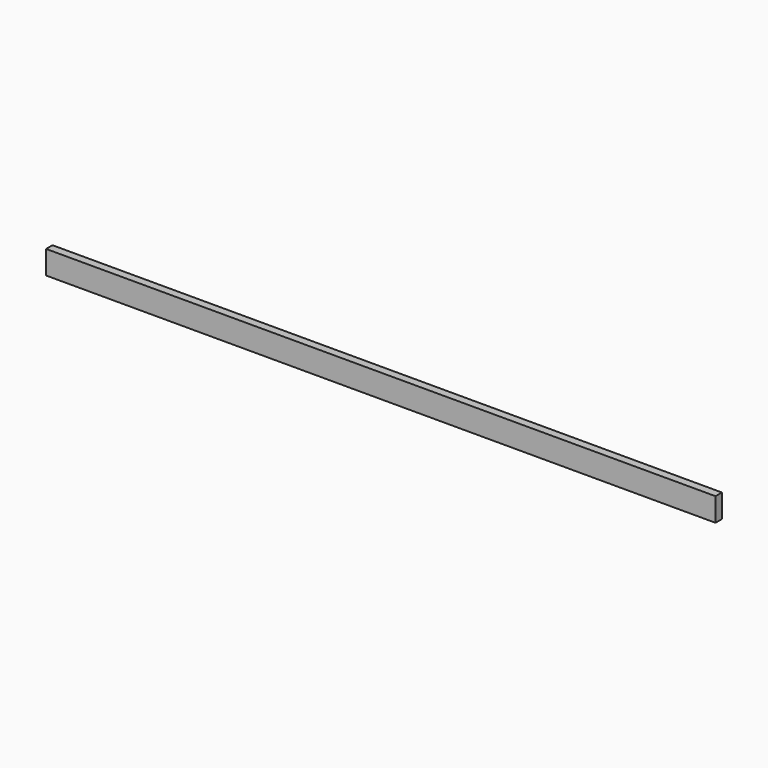
from build123d import *

# Parameters (mm, degrees)
F0_W     = 1000
F0_H     = 35
F1_DEPTH = 12


# Not quite as in the source:
# - a feature names something its author has since deleted; it is built from what else it names


with BuildPart() as f1:
    # F0 (on Front) → F1 (new body)
    with BuildSketch(Plane.XZ):
        with Locations((500, 17.5)):
            Rectangle(F0_W, F0_H)
    extrude(amount=F1_DEPTH)


solid = f1.part
